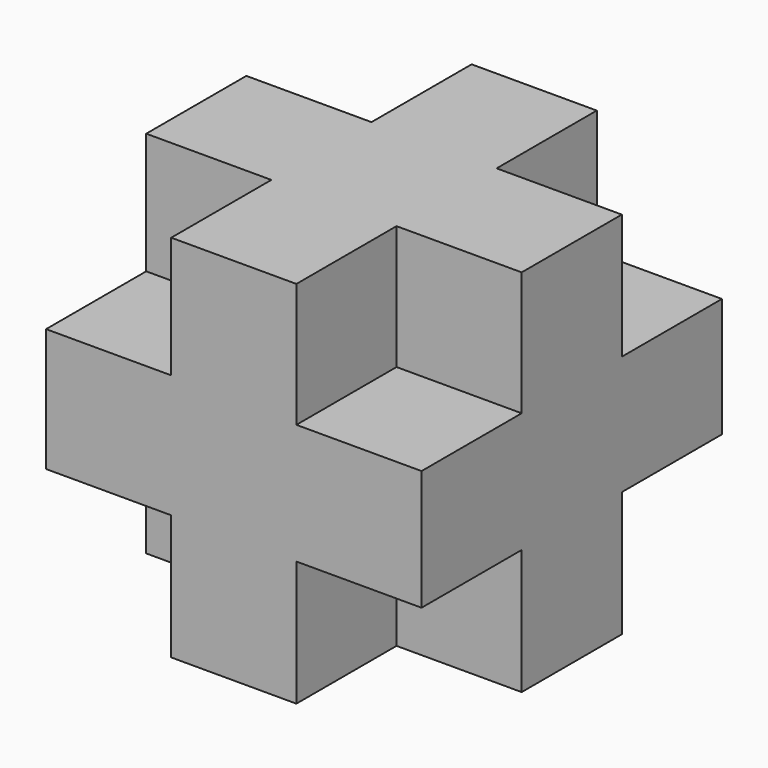
from build123d import *

# Parameters (mm, degrees)
F0_W      = 152.4
F0_H      = 149.9905144195
F1_DEPTH  = 152.4
F2_W      = 50.8
F2_H      = 49.1875803169
F3_DEPTH  = 50.8
F4_W      = 50.8
F4_H      = 50.3492622576
F5_DEPTH  = 50.8
F6_W      = 50.8
F6_H      = 50.8
F7_DEPTH  = 343
F8_W      = 50.8
F8_H      = 50.8
F9_DEPTH  = 50.8
F10_W     = 50.8
F10_H     = 50.8
F11_DEPTH = 50.8
F12_W     = 50.8
F12_H     = 50.8
F13_DEPTH = 50.8


# Not quite as in the source:
# - an extrude ends at something that could not be found from the text; its depth is read off the source's solid
# - a feature names something its author has since deleted; it is built from what else it names


with BuildPart() as f1:
    # F0 (on Front) → F1 (new body)
    with BuildSketch(Plane.XZ):
        with Locations((3.4536700696, 3.1658634543)):
            Rectangle(F0_W, F0_H)
    extrude(amount=F1_DEPTH)

    # F2 (on face) → F3 (cut)
    with BuildSketch(Plane.XZ.offset(152.4)):
        with Locations((-47.3463299304, 53.5673305057)):
            Rectangle(F2_W, F2_H)
    extrude(amount=-F3_DEPTH, mode=Mode.SUBTRACT)

    # F4 (on face) → F5 (cut)
    with BuildSketch(Plane.XZ.offset(152.4)):
        with Locations((54.2536700696, 52.9864895353)):
            Rectangle(F4_W, F4_H)
    extrude(amount=-F5_DEPTH, mode=Mode.SUBTRACT)

    # F6 (on face) → F7 (cut, through all)
    with BuildSketch(Plane.XZ.offset(152.4)):
        with Locations((-47.3463299304, -46.4293937554)):
            Rectangle(F6_W, F6_H)
    extrude(amount=F7_DEPTH, mode=Mode.SUBTRACT)

    # F8 (on face) → F9 (cut)
    with BuildSketch(Plane(origin=(0, 0, 0), x_dir=(-1, 0, 0), z_dir=(0, 1, 0))):
        with Locations((-54.2536700696, -46.4293937554)):
            Rectangle(F8_W, F8_H)
        with Locations((47.3463299304, -46.4293937554)):
            Rectangle(F8_W, F8_H)
    extrude(amount=-F9_DEPTH, mode=Mode.SUBTRACT)

    # F10 (on face) → F11 (cut)
    with BuildSketch(Plane(origin=(0, 0, -71.8293937554), x_dir=(1, 0, 0), z_dir=(0, 0, -1))):
        with Locations((-47.3463299304, 127)):
            Rectangle(F10_W, F10_H)
        with Locations((54.2536700696, 127)):
            Rectangle(F10_W, F10_H)
    extrude(amount=-F11_DEPTH, mode=Mode.SUBTRACT)

    # F12 (on face) → F13 (cut)
    with BuildSketch(Plane.XY.offset(78.1611206641)):
        with Locations((-47.3463299304, -25.4)):
            Rectangle(F12_W, F12_H)
        with Locations((54.2536700696, -25.4)):
            Rectangle(F12_W, F12_H)
    extrude(amount=-F13_DEPTH, mode=Mode.SUBTRACT)


solid = f1.part
